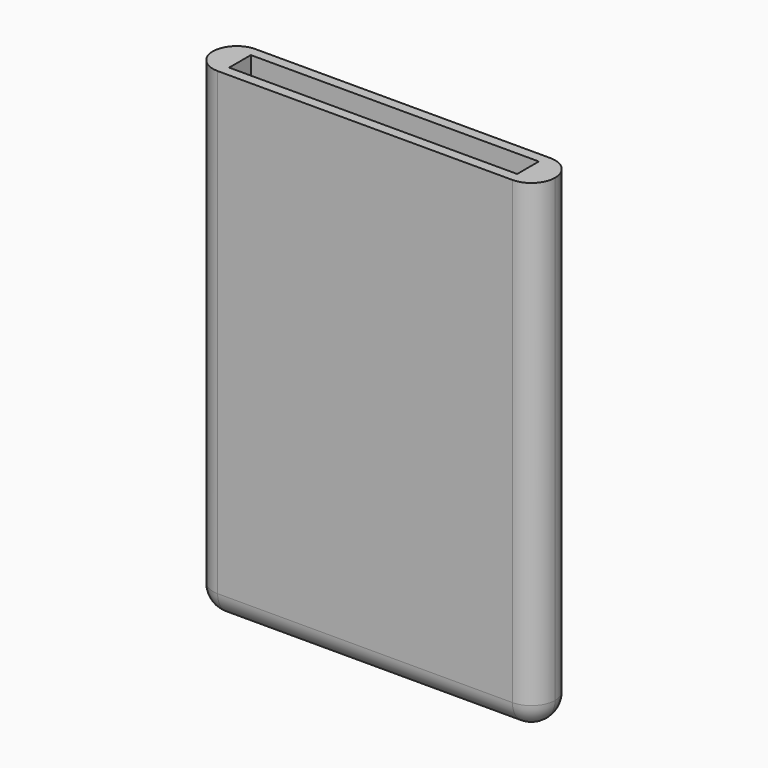
from build123d import *

# Parameters (mm, degrees)
F1_DEPTH  = 6.35
F2_DEPTH  = 1.27
F3_W      = 1.27
F3_H      = 85.6234
F4_DEPTH  = 54.0004
F5_DEPTH  = 1.27
F6_W      = 1.27
F6_H      = 85.6234
F7_DEPTH  = 54.0004
F8_R      = 4.44499
F9_DEPTH  = 0.635
F10_DEPTH = 0.635


# Not quite as in the source:
# - a fillet or chamfer is up to 0.001 mm smaller than in the source, because OpenCascade refuses the exact size


with BuildPart() as f1:
    # F0 (on Front) → F1 (new body)
    with BuildSketch(Plane.XZ):
        Polygon((54.0004, 0), (0, 0), (0, 85.6234), (-5.08, 85.6234), (-5.08, 0), (-5.08, -5.08), (0, -5.08), (54.0004, -5.08), (59.0804, -5.08), (59.0804, 0), (59.0804, 85.6234), (54.0004, 85.6234), align=None)
    extrude(amount=F1_DEPTH)

    # F2 (add): a face of the model
    f2_faces = [f1.faces().sort_by_distance(p)[0] for p in [
        (27.0002, -6.35, -3.9689795817),
    ]]
    extrude(f2_faces, amount=F2_DEPTH)

    # F3 (on face) → F4 (join)
    with BuildSketch(Plane(origin=(54.0004, 0, 0), x_dir=(0, -1, 0), z_dir=(-1, 0, 0))):
        with Locations((6.985, 42.8117)):
            Rectangle(F3_W, F3_H)
    extrude(amount=F4_DEPTH)

    # F5 (add): a face of the model
    f5_faces = [f1.faces().sort_by_distance(p)[0] for p in [
        (27.0002, 0, -3.9689795817),
    ]]
    extrude(f5_faces, amount=F5_DEPTH)

    # F6 (on face) → F7 (join)
    with BuildSketch(Plane(origin=(54.0004, 0, 0), x_dir=(0, -1, 0), z_dir=(-1, 0, 0))):
        with Locations((-0.635, 42.8117)):
            Rectangle(F6_W, F6_H)
    extrude(amount=F7_DEPTH)

    # F8 (radius 4.445 in the source; OpenCascade refuses exactly that, so slightly less here)
    f8_edges = [f1.edges().sort_by_distance(p)[0] for p in [
        (-5.08, -7.62, 40.2717),
        (-5.08, 1.27, 40.2717),
        (59.0804, 1.27, 40.2717),
        (59.0804, -7.62, 40.2717),
        (-5.08, -3.175, -5.08),
        (27.0002, 1.27, -5.08),
        (27.0002, -7.62, -5.08),
        (59.0804, -3.175, -5.08),
    ]]
    fillet(f8_edges, radius=F8_R)

    # F9 (add): a face of the model
    f9_faces = [f1.faces().sort_by_distance(p)[0] for p in [
        (27.0002, 0, 42.8117),
    ]]
    extrude(f9_faces, amount=F9_DEPTH)

    # F10 (add): a face of the model
    f10_faces = [f1.faces().sort_by_distance(p)[0] for p in [
        (27.0002, -6.35, 42.8117),
    ]]
    extrude(f10_faces, amount=F10_DEPTH)


solid = f1.part
